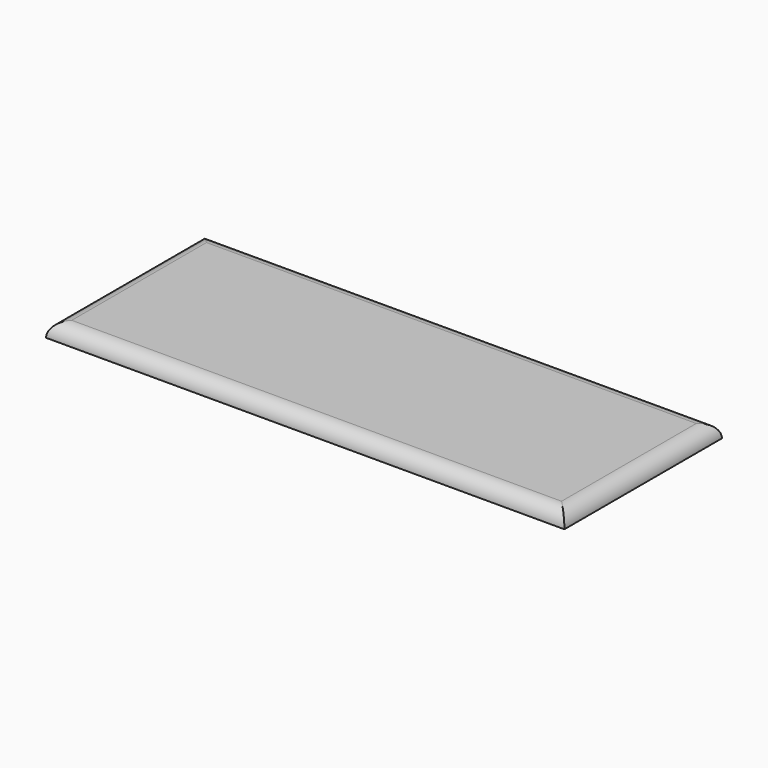
from build123d import *

# Parameters (mm, degrees)
F0_W     = 181.7570477724
F0_H     = 69.0473541617
F1_DEPTH = 5
F2_R     = 4.99999


# Not quite as in the source:
# - a fillet or chamfer is up to 0.001 mm smaller than in the source, because OpenCascade refuses the exact size


with BuildPart() as f1:
    # F0 (on Top) → F1 (new body)
    with BuildSketch(Plane.XY):
        Rectangle(F0_W, F0_H)
    extrude(amount=F1_DEPTH)

    # F2 (radius 5 in the source; OpenCascade refuses exactly that, so slightly less here)
    f2_edges = [f1.edges().sort_by_distance(p)[0] for p in [
        (0, -34.523677, 5),
        (-90.878524, 0, 5),
        (0, 34.523677, 5),
        (90.878524, 0, 5),
    ]]
    fillet(f2_edges, radius=F2_R)


solid = f1.part
